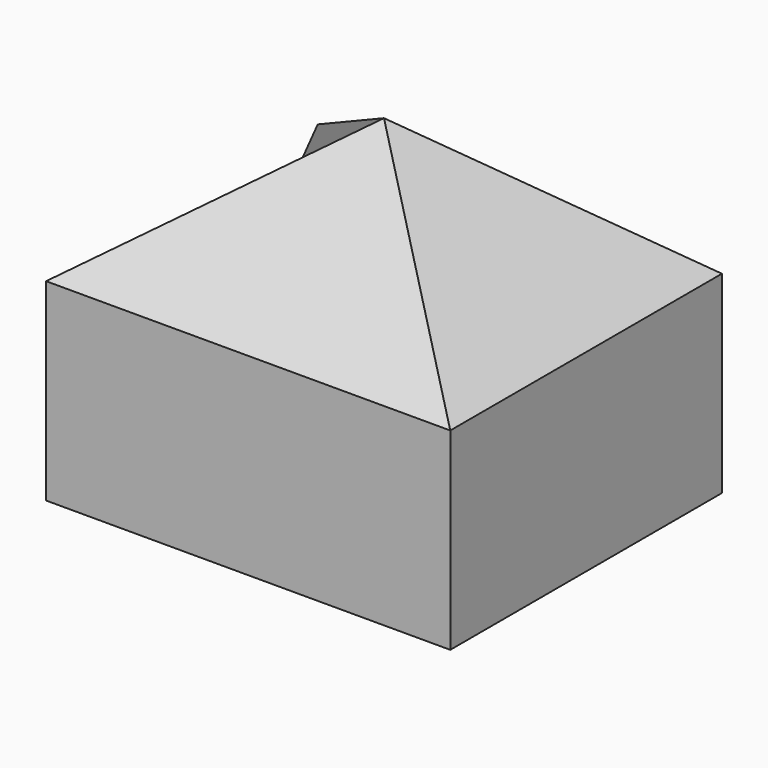
from build123d import *

# Parameters (mm, degrees)
F0_W     = 73.3171850443
F0_H     = 60.4678094387
F1_DEPTH = 30.8
F3_DEPTH = 61.601
F5_DEPTH = 73.3181850443


# Not quite as in the source:
# - a feature of the source that left no trace in its solid (it failed there, or was rolled back) is left out


with BuildPart() as f1:
    # F0 (on Front) → F1 (new body, symmetric)
    with BuildSketch(Plane.XZ):
        Rectangle(F0_W, F0_H)
    extrude(amount=F1_DEPTH, both=True)

    # F2 (on face) → F3 (cut, through all)
    with BuildSketch(Plane.XZ.offset(30.8)):
        Polygon((-36.6585925221, 30.2339047194), (-36.6585925221, 4.7981617972), (0, 30.2339047194), align=None)
        Polygon((36.6585925221, 30.2339047194), (0, 30.2339047194), (36.6585925221, 4.7981617972), align=None)
    extrude(amount=-F3_DEPTH, mode=Mode.SUBTRACT)

    # F4 (on face) → F5 (cut, through all)
    with BuildSketch(Plane(origin=(-36.6585925221, 0, 0), x_dir=(0, -1, 0), z_dir=(-1, 0, 0))):
        Polygon((0, 30.2339047194), (-30.8, 30.2339047194), (-30.8, 4.7981617972), align=None)
        Polygon((30.8, 30.2339047194), (0, 30.2339047194), (30.8, 4.7981617972), align=None)
    extrude(amount=-F5_DEPTH, mode=Mode.SUBTRACT)

    # F10: sweep along a path in F9
    with BuildLine(Plane(origin=(-9.9452522809, 6.8577617895, 6.0293064075), x_dir=(-0.4343419548, -0.8613999118, 0.2633196883), z_dir=(-0.7366055839, 0.5079273491, 0.4465669287))) as f10_path:
        Line((7.9611823679, -9.5022734797), (43.7169324882, -14.9015133699))
    # F6 (on Front) → F10 (sweep, cut)
    with BuildSketch(Plane.XZ):
        Polygon((-36.6585925221, 4.7981617972), (-36.6585925221, -30.2339047194), (0, 30.2339047194), align=None)
    sweep(path=f10_path.line, mode=Mode.SUBTRACT)

    # F11: F1 across plane


with BuildPart() as f1_1:
    add(f1.part)
    add(f1.part.mirror(Plane.XZ), mode=Mode.INTERSECT)


solid = f1_1.part
